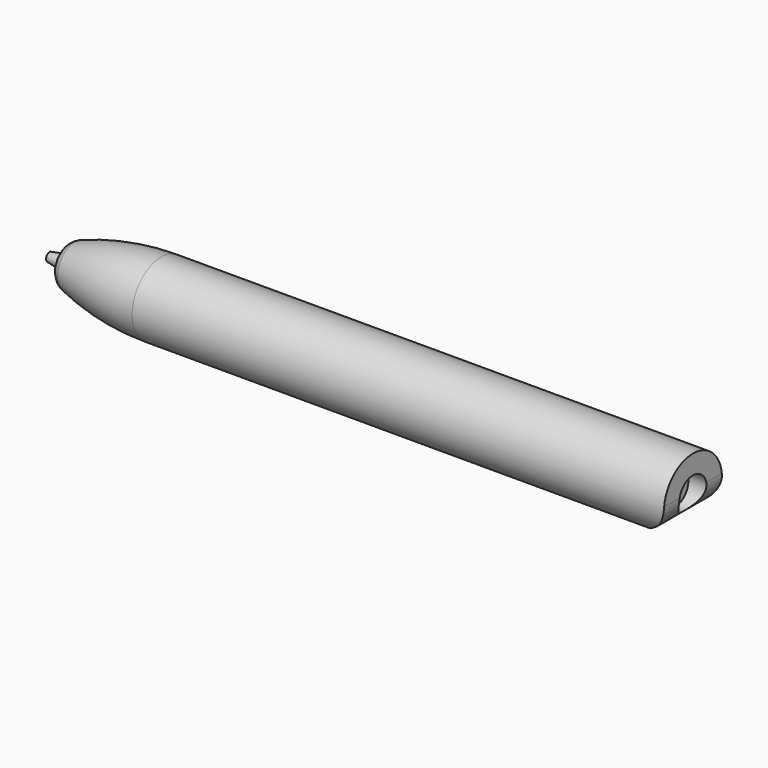
from build123d import *

# Parameters (mm, degrees)
F5_DEPTH    = 25.4
F7_DEPTH    = 12.7
F8_T1_DEPTH = 17.0147141114
F8_T3_DEPTH = 17.0147141114
F9_SIZE2    = 0.447870531
F9_SIZE     = 2.54
F10_R       = 2.54


# Not quite as in the source:
# - a fillet or chamfer that OpenCascade refuses, or shapes differently, is made with other operations: its cross-section is extruded or revolved along the edge and cut away or added


with BuildPart() as f1:
    # F0 (on Front) → F1 (revolve)
    with BuildSketch(Plane.XZ):
        Polygon((-109.4232, 0), (0, 0), (0, 2.9845), (-90.678, 2.9845), (-90.678, 2.2606), (-100.7872, 2.2606), (-100.7872, 1.5494), (-100.7872, 1.2065), (-109.4232, 1.2065), align=None)
    revolve(axis=Axis((-54.7116, 0, 0), (1, 0, 0)))


with BuildPart() as f3:
    # F2 (on Front) → F3 (revolve)
    with BuildSketch(Plane.XZ):
        with BuildLine():
            Line((0, 6.35), (-89.8901687584, 6.35))
            ThreePointArc((-89.8901687584, 6.35), (-98.4389065262, 5.5354684697), (-106.68, 3.1211865076))
            Line((-106.68, 3.1211865076), (-106.68, 0))
            Line((-106.68, 0), (0, 0))
            Line((0, 0), (3.175, 0))
            Line((3.175, 0), (3.175, 6.35))
            Line((3.175, 6.35), (0, 6.35))
        make_face()
    revolve(axis=Axis((-53.34, 0, 0), (1, 0, 0)))

    # F4: cut F1
    add(f1.part, mode=Mode.SUBTRACT)

    # F5 (cut): a face of the model
    f5_faces = [f1.part.faces().sort_by_distance(p)[0] for p in [
        (0, 0, 0),
    ]]
    extrude(f5_faces, amount=F5_DEPTH, mode=Mode.SUBTRACT)

    # F6 (on Front) → F7 (cut, symmetric)
    with BuildSketch(Plane.XZ):
        Polygon((34.4975971024, 19.9667225742), (-4.445, -7.3011774743), (-4.445, -25.4), (34.4975971024, -25.4), align=None)
    extrude(amount=F7_DEPTH, both=True, mode=Mode.SUBTRACT)

    # F8: fillet of radius 5.08 on 2 edges, made by hand

    # F8_s2 → F8_t1 (cut)
    with BuildSketch(Plane.XZ.offset(-4.3653893316)):
        with BuildLine():
            ThreePointArc((3.175, 0.6788845836), (2.6010150325, -1.6667983716), (1.0087682967, -3.4824078013))
            Line((1.0087682967, -3.4824078013), (3.175, -1.9655960332))
            Line((3.175, -1.9655960332), (3.175, 0.6788845836))
        make_face()
    extrude(amount=F8_T1_DEPTH, mode=Mode.SUBTRACT)

    # F8_s4 → F8_t3 (cut)
    with BuildSketch(Plane.XZ.offset(-12.6493247798)):
        with BuildLine():
            ThreePointArc((3.175, 0.6788845836), (2.6010150325, -1.6667983716), (1.0087682967, -3.4824078013))
            Line((1.0087682967, -3.4824078013), (3.175, -1.9655960332))
            Line((3.175, -1.9655960332), (3.175, 0.6788845836))
        make_face()
    extrude(amount=F8_T3_DEPTH, mode=Mode.SUBTRACT)

    # F10
    f10_edges = [f3.edges().sort_by_distance(p)[0] for p in [
        (-106.68, 0, -3.121187),
    ]]
    fillet(f10_edges, radius=F10_R)


with BuildPart() as f1_1:
    add(f1.part)

    # F9
    f9_edges = [f1_1.edges().sort_by_distance(p)[0] for p in [
        (-109.4232, 0, -1.2065),
    ]]
    chamfer(f9_edges, length=F9_SIZE, length2=F9_SIZE2)


solid = Compound([f3.part, f1_1.part])
